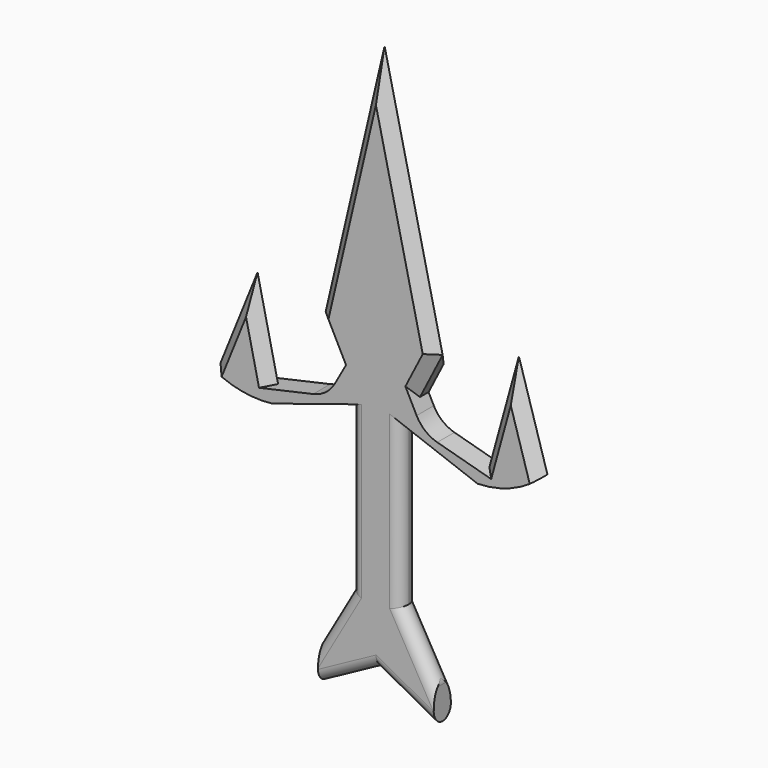
from build123d import *

# Parameters (mm, degrees)
F1_DEPTH      = 3.302
F2_SIZE       = 1.65099
F3_R          = 5.08
F4_T1_DEPTH   = 5.391144251
F4_T6_DEPTH   = 33.5393354473
F4_T12_DEPTH  = 33.5393354473
F4_T18_DEPTH  = 33.5393354473
F4_T24_DEPTH  = 33.5393354473
F4_T30_DEPTH  = 18.415
F4_T35_DEPTH  = 18.415
F4_T40_DEPTH  = 18.415
F4_T45_DEPTH  = 18.415
F4_T50_DEPTH  = 18.415
F4_T55_DEPTH  = 18.415
F4_T60_DEPTH  = 18.415
F4_T65_DEPTH  = 18.415
F4_T71_DEPTH  = 18.415
F4_T75_DEPTH  = 33.5393354473
F4_T82_DEPTH  = 33.5393354473
F4_T86_DEPTH  = 18.415
F4_T93_DEPTH  = 18.415
F4_T97_DEPTH  = 33.5393354473
F4_T104_DEPTH = 33.5393354473
F4_T108_DEPTH = 18.415
F4_T115_DEPTH = 18.415
F4_T119_DEPTH = 18.415
F4_T126_DEPTH = 18.415
F4_T130_DEPTH = 18.415


# Not quite as in the source:
# - a fillet or chamfer that OpenCascade refuses, or shapes differently, is made with other operations: its cross-section is extruded or revolved along the edge and cut away or added
# - a fillet or chamfer is up to 0.001 mm smaller than in the source, because OpenCascade refuses the exact size


with BuildPart() as f1:
    # F0 (on Front) → F1 (new body)
    with BuildSketch(Plane.XZ):
        Polygon((-8.9293484636, -27.2495914251), (-8.9293484636, -32.5835914251), (0, -27.7367021117), (8.9302421297, -32.5819446757), (8.7977098301, -27.2495914251), (3.7441806833, -18.4355433674), (-3.8758193167, -18.4355433674), align=None)
        Polygon((-3.8758193167, 6.8487920798), (-3.8758193167, -18.4355433674), (3.7441806833, -18.4355433674), (3.7441806833, 6.8487920798), (5.4475756045, 10.1900669473), (8.9355429432, 17.0318494737), (0, 55.9675879776), (-9.0671815766, 17.0318494737), (-5.5792142379, 10.1900669473), align=None)
        Polygon((-15.9811842538, 3.0082010134), (-3.8758193167, 6.8487920798), (-5.5792142379, 10.1900669473), (-7.4475542642, 6.8487920798), (-16.3927144946, 4.8489290213), align=None)
        Polygon((5.4475756045, 10.1900669473), (3.7441806833, 6.8487920798), (15.648767343, 2.4249005283), (16.1309282999, 4.1770842273), (7.269941736, 6.61542546), align=None)
        with BuildLine():
            ThreePointArc((-25.2471491773, 4.8381724725), (-20.7595085955, 3.1872557237), (-15.9811842538, 3.0082010134))
            Line((-15.9811842538, 3.0082010134), (-16.3927144946, 4.8489290213))
            Line((-16.3927144946, 4.8489290213), (-19.5505233946, 18.973449431))
            Line((-19.5505233946, 18.973449431), (-25.2471491773, 4.8381724725))
        make_face()
        with BuildLine():
            Line((16.1309282999, 4.1770842273), (15.648767343, 2.4249005283))
            ThreePointArc((15.648767343, 2.4249005283), (20.6670070739, 3.4448326602), (25.0641160129, 6.0694134893))
            Line((25.0641160129, 6.0694134893), (20.6670070739, 20.6612959236))
            Line((20.6670070739, 20.6612959236), (16.1309282999, 4.1770842273))
        make_face()
    extrude(amount=F1_DEPTH)

    # F2 (size 1.651 in the source; OpenCascade refuses exactly that, so slightly less here)
    f2_edges = [f1.edges().sort_by_distance(p)[0] for p in [
        (4.467771, -3.302, 36.499719),
        (-4.533591, -3.302, 36.499719),
        (18.398968, -3.302, 12.41919),
        (22.865562, -3.302, 13.365355),
        (-22.398836, -3.302, 11.905811),
        (-17.971619, -3.302, 11.911189),
        (18.398968, 0, 12.41919),
        (22.865562, 0, 13.365355),
        (-22.398836, 0, 11.905811),
        (-17.971619, 0, 11.911189),
        (7.191559, -3.302, 13.610958),
        (-7.323198, -3.302, 13.610958),
        (4.467771, 0, 36.499719),
        (-4.533591, 0, 36.499719),
    ]]
    chamfer(f2_edges, length=F2_SIZE)

    # F3
    f3_edges = [f1.edges().sort_by_distance(p)[0] for p in [
        (-7.447554, -1.651, 6.848792),
        (7.269942, -1.651, 6.615425),
    ]]
    fillet(f3_edges, radius=F3_R)

    # F4: fillet of radius 1.651 on 13 edges, made by hand

    # F4_s2 → F4_t1 (cut)
    with BuildSketch(Plane.XZ.offset(-1.0445721255)):
        with BuildLine():
            ThreePointArc((8.5898840158, -26.8871146962), (8.7475827705, -27.2636114555), (8.8080914983, -27.6672912803))
            Line((8.8080914983, -27.6672912803), (8.7977098301, -27.2495914251))
            Line((8.7977098301, -27.2495914251), (8.5898840158, -26.8871146962))
        make_face()
    extrude(amount=F4_T1_DEPTH, mode=Mode.SUBTRACT)


with BuildPart() as f4_tool4:
    # F4_s5 → F4_t6 (new body)
    with BuildSketch(Plane.XY.offset(10.9762920798)):
        with BuildLine():
            ThreePointArc((-3.8758193167, -1.651), (-3.3922526125, -2.8184332957), (-2.2248193167, -3.302))
            Line((-2.2248193167, -3.302), (-3.8758193167, -3.302))
            Line((-3.8758193167, -3.302), (-3.8758193167, -1.651))
        make_face()
    extrude(amount=-F4_T6_DEPTH)

    split(bisect_by=Plane(origin=(5.03803687, 0, -2.888555406), x_dir=(0, 1, 0), z_dir=(-0.8675244151, 0, 0.4973946011)), keep=Keep.TOP)

    split(bisect_by=Plane(origin=(-2.3286084058, 0, 7.3396657076), x_dir=(0, 1, 0), z_dir=(0.3024087454, 0, -0.9531783415)), keep=Keep.TOP)


with BuildPart() as f1_1:
    add(f1.part)

    # F4_t3: cut F4_tool4
    add(f4_tool4.part, mode=Mode.SUBTRACT)


with BuildPart() as f4_tool10:
    # F4_s11 → F4_t12 (new body)
    with BuildSketch(Plane.XY.offset(-22.5630433674)):
        with BuildLine():
            ThreePointArc((3.7441806833, -1.651), (3.260613979, -2.8184332957), (2.0931806833, -3.302))
            Line((2.0931806833, -3.302), (3.7441806833, -3.302))
            Line((3.7441806833, -3.302), (3.7441806833, -1.651))
        make_face()
    extrude(amount=F4_T12_DEPTH)

    split(bisect_by=Plane(origin=(2.6905919195, 0, 7.2403186875), x_dir=(0, 1, 0), z_dir=(-0.3483379174, 0, -0.9373690283)), keep=Keep.TOP)

    split(bisect_by=Plane(origin=(-5.1371079227, 0, -2.9453577344), x_dir=(0, 1, 0), z_dir=(0.8675244151, 0, 0.4973946011)), keep=Keep.TOP)


with BuildPart() as f1_2:
    add(f1_1.part)

    # F4_t9: cut F4_tool10
    add(f4_tool10.part, mode=Mode.SUBTRACT)


with BuildPart() as f4_tool16:
    # F4_s17 → F4_t18 (new body)
    with BuildSketch(Plane.XY.offset(10.9762920798)):
        with BuildLine():
            ThreePointArc((-2.2248193167, 0), (-3.3922526125, -0.4835667043), (-3.8758193167, -1.651))
            Line((-3.8758193167, -1.651), (-3.8758193167, 0))
            Line((-3.8758193167, 0), (-2.2248193167, 0))
        make_face()
    extrude(amount=-F4_T18_DEPTH)

    split(bisect_by=Plane(origin=(5.03803687, 0, -2.888555406), x_dir=(0, 1, 0), z_dir=(-0.8675244151, 0, 0.4973946011)), keep=Keep.TOP)

    split(bisect_by=Plane(origin=(-2.3286084058, 0, 7.3396657076), x_dir=(0, 1, 0), z_dir=(0.3024087454, 0, -0.9531783415)), keep=Keep.TOP)


with BuildPart() as f1_3:
    add(f1_2.part)

    # F4_t15: cut F4_tool16
    add(f4_tool16.part, mode=Mode.SUBTRACT)


with BuildPart() as f4_tool22:
    # F4_s23 → F4_t24 (new body)
    with BuildSketch(Plane.XY.offset(-22.5630433674)):
        with BuildLine():
            ThreePointArc((2.0931806833, 0), (3.260613979, -0.4835667043), (3.7441806833, -1.651))
            Line((3.7441806833, -1.651), (3.7441806833, 0))
            Line((3.7441806833, 0), (2.0931806833, 0))
        make_face()
    extrude(amount=F4_T24_DEPTH)

    split(bisect_by=Plane(origin=(2.6905919195, 0, 7.2403186875), x_dir=(0, 1, 0), z_dir=(-0.3483379174, 0, -0.9373690283)), keep=Keep.TOP)

    split(bisect_by=Plane(origin=(-5.1371079227, 0, -2.9453577344), x_dir=(0, 1, 0), z_dir=(0.8675244151, 0, 0.4973946011)), keep=Keep.TOP)


with BuildPart() as f1_4:
    add(f1_3.part)

    # F4_t21: cut F4_tool22
    add(f4_tool22.part, mode=Mode.SUBTRACT)


with BuildPart() as f4_tool28:
    # F4_s29 → F4_t30 (new body)
    with BuildSketch(Plane(origin=(-6.8608599708, 0, -11.966280938), x_dir=(0, 1, 0), z_dir=(-0.4973946011, 0, -0.8675244151))):
        with BuildLine():
            ThreePointArc((0, 7.4583718528), (-0.4835667043, 6.2909385571), (-1.651, 5.8073718528))
            Line((-1.651, 5.8073718528), (0, 5.8073718528))
            Line((0, 5.8073718528), (0, 7.4583718528))
        make_face()
    extrude(amount=F4_T30_DEPTH)

    split(bisect_by=Plane.YZ.offset(-3.8758193167), keep=Keep.BOTTOM)


with BuildPart() as f1_5:
    add(f1_4.part)

    # F4_t27: cut F4_tool28
    add(f4_tool28.part, mode=Mode.SUBTRACT)


with BuildPart() as f4_tool33:
    # F4_s34 → F4_t35 (new body)
    with BuildSketch(Plane(origin=(-6.8608599708, 0, -11.966280938), x_dir=(0, 1, 0), z_dir=(-0.4973946011, 0, -0.8675244151))):
        with BuildLine():
            ThreePointArc((-1.651, 5.8073718528), (-2.8184332957, 6.2909385571), (-3.302, 7.4583718528))
            Line((-3.302, 7.4583718528), (-3.302, 5.8073718528))
            Line((-3.302, 5.8073718528), (-1.651, 5.8073718528))
        make_face()
    extrude(amount=F4_T35_DEPTH)

    split(bisect_by=Plane.YZ.offset(-3.8758193167), keep=Keep.BOTTOM)


with BuildPart() as f1_6:
    add(f1_5.part)

    # F4_t32: cut F4_tool33
    add(f4_tool33.part, mode=Mode.SUBTRACT)


with BuildPart() as f4_tool38:
    # F4_s39 → F4_t40 (new body)
    with BuildSketch(Plane(origin=(-24.1861080645, 0, -13.1283250048), x_dir=(0, 1, 0), z_dir=(0.8788728803, 0, 0.4770560348))):
        with BuildLine():
            ThreePointArc((0, -22.7260352741), (-0.4835667043, -23.8934685698), (-1.651, -24.3770352741))
            Line((-1.651, -24.3770352741), (0, -24.3770352741))
            Line((0, -24.3770352741), (0, -22.7260352741))
        make_face()
    extrude(amount=F4_T40_DEPTH)

    split(bisect_by=Plane(origin=(-11.6264241962, 0, -21.4286037908), x_dir=(0, 1, 0), z_dir=(-0.4768939532, 0, -0.8789608395)), keep=Keep.TOP)


with BuildPart() as f1_7:
    add(f1_6.part)

    # F4_t37: cut F4_tool38
    add(f4_tool38.part, mode=Mode.SUBTRACT)


with BuildPart() as f4_tool43:
    # F4_s44 → F4_t45 (new body)
    with BuildSketch(Plane(origin=(-24.1861080645, 0, -13.1283250048), x_dir=(0, 1, 0), z_dir=(0.8788728803, 0, 0.4770560348))):
        with BuildLine():
            ThreePointArc((-1.651, -24.3770352741), (-2.8184332957, -23.8934685698), (-3.302, -22.7260352741))
            Line((-3.302, -22.7260352741), (-3.302, -24.3770352741))
            Line((-3.302, -24.3770352741), (-1.651, -24.3770352741))
        make_face()
    extrude(amount=F4_T45_DEPTH)

    split(bisect_by=Plane(origin=(-11.6264241962, 0, -21.4286037908), x_dir=(0, 1, 0), z_dir=(-0.4768939532, 0, -0.8789608395)), keep=Keep.TOP)


with BuildPart() as f1_8:
    add(f1_7.part)

    # F4_t42: cut F4_tool43
    add(f4_tool43.part, mode=Mode.SUBTRACT)


with BuildPart() as f4_tool48:
    # F4_s49 → F4_t50 (new body)
    with BuildSketch(Plane(origin=(15.9878139687, 0, -27.8849407141), x_dir=(0, 1, 0), z_dir=(-0.4973946011, 0, 0.8675244151))):
        with BuildLine():
            ThreePointArc((-1.651, 5.9215715813), (-2.8184332957, 6.4051382856), (-3.302, 7.5725715813))
            Line((-3.302, 7.5725715813), (-3.302, 5.9215715813))
            Line((-3.302, 5.9215715813), (-1.651, 5.9215715813))
        make_face()
    extrude(amount=F4_T50_DEPTH)

    split(bisect_by=Plane.YZ.offset(3.7441806833), keep=Keep.TOP)


with BuildPart() as f1_9:
    add(f1_8.part)

    # F4_t47: cut F4_tool48
    add(f4_tool48.part, mode=Mode.SUBTRACT)


with BuildPart() as f4_tool53:
    # F4_s54 → F4_t55 (new body)
    with BuildSketch(Plane(origin=(15.9878139687, 0, -27.8849407141), x_dir=(0, 1, 0), z_dir=(-0.4973946011, 0, 0.8675244151))):
        with BuildLine():
            ThreePointArc((0, 7.5725715813), (-0.4835667043, 6.4051382856), (-1.651, 5.9215715813))
            Line((-1.651, 5.9215715813), (0, 5.9215715813))
            Line((0, 5.9215715813), (0, 7.5725715813))
        make_face()
    extrude(amount=F4_T55_DEPTH)

    split(bisect_by=Plane.YZ.offset(3.7441806833), keep=Keep.TOP)


with BuildPart() as f1_10:
    add(f1_9.part)

    # F4_t52: cut F4_tool53
    add(f4_tool53.part, mode=Mode.SUBTRACT)


with BuildPart() as f4_tool58:
    # F4_s59 → F4_t60 (new body)
    with BuildSketch(Plane(origin=(7.998513331, 0, -4.3397185292), x_dir=(0, 1, 0), z_dir=(0.8789608395, 0, -0.4768939532))):
        with BuildLine():
            ThreePointArc((0, -22.7284749742), (-0.4835667043, -23.8959082699), (-1.651, -24.3794749742))
            Line((-1.651, -24.3794749742), (0, -24.3794749742))
            Line((0, -24.3794749742), (0, -22.7284749742))
        make_face()
    extrude(amount=F4_T60_DEPTH)

    split(bisect_by=Plane(origin=(11.6292117876, 0, -21.4243152038), x_dir=(0, 1, 0), z_dir=(0.4770560348, 0, -0.8788728803)), keep=Keep.TOP)


with BuildPart() as f1_11:
    add(f1_10.part)

    # F4_t57: cut F4_tool58
    add(f4_tool58.part, mode=Mode.SUBTRACT)


with BuildPart() as f4_tool63:
    # F4_s64 → F4_t65 (new body)
    with BuildSketch(Plane(origin=(7.998513331, 0, -4.3397185292), x_dir=(0, 1, 0), z_dir=(0.8789608395, 0, -0.4768939532))):
        with BuildLine():
            ThreePointArc((-1.651, -24.3794749742), (-2.8184332957, -23.8959082699), (-3.302, -22.7284749742))
            Line((-3.302, -22.7284749742), (-3.302, -24.3794749742))
            Line((-3.302, -24.3794749742), (-1.651, -24.3794749742))
        make_face()
    extrude(amount=F4_T65_DEPTH)

    split(bisect_by=Plane(origin=(11.6292117876, 0, -21.4243152038), x_dir=(0, 1, 0), z_dir=(0.4770560348, 0, -0.8788728803)), keep=Keep.TOP)


with BuildPart() as f1_12:
    add(f1_11.part)

    # F4_t62: cut F4_tool63
    add(f4_tool63.part, mode=Mode.SUBTRACT)


with BuildPart() as f4_tool69:
    # F4_s70 → F4_t71 (new body)
    with BuildSketch(Plane(origin=(-6.8608599708, 0, -11.966280938), x_dir=(0, 1, 0), z_dir=(-0.4973946011, 0, -0.8675244151))):
        with BuildLine():
            ThreePointArc((-1.651, 5.8073718528), (-2.8184332957, 6.2909385571), (-3.302, 7.4583718528))
            Line((-3.302, 7.4583718528), (-3.302, 5.8073718528))
            Line((-3.302, 5.8073718528), (-1.651, 5.8073718528))
        make_face()
    extrude(amount=F4_T71_DEPTH)

    split(bisect_by=Plane.YZ.offset(-3.8758193167), keep=Keep.TOP)


with BuildPart() as f4_tool73:
    # F4_s74 → F4_t75 (new body)
    with BuildSketch(Plane.XY.offset(10.9762920798)):
        with BuildLine():
            ThreePointArc((-3.8758193167, -1.651), (-3.3922526125, -2.8184332957), (-2.2248193167, -3.302))
            Line((-2.2248193167, -3.302), (-3.8758193167, -3.302))
            Line((-3.8758193167, -3.302), (-3.8758193167, -1.651))
        make_face()
    extrude(amount=-F4_T75_DEPTH)

    split(bisect_by=Plane(origin=(5.03803687, 0, -2.888555406), x_dir=(0, 1, 0), z_dir=(0.8675244151, 0, -0.4973946011)), keep=Keep.TOP)


with BuildPart() as f4_tool69_1:
    add(f4_tool69.part)

    # F4_t77: intersect F4_tool73
    add(f4_tool73.part, mode=Mode.INTERSECT)


with BuildPart() as f1_13:
    add(f1_12.part)

    # F4_t67: cut F4_tool69
    add(f4_tool69_1.part, mode=Mode.SUBTRACT)


with BuildPart() as f4_tool80:
    # F4_s81 → F4_t82 (new body)
    with BuildSketch(Plane.XY.offset(-22.5630433674)):
        with BuildLine():
            ThreePointArc((3.7441806833, -1.651), (3.260613979, -2.8184332957), (2.0931806833, -3.302))
            Line((2.0931806833, -3.302), (3.7441806833, -3.302))
            Line((3.7441806833, -3.302), (3.7441806833, -1.651))
        make_face()
    extrude(amount=F4_T82_DEPTH)

    split(bisect_by=Plane(origin=(-5.1371079227, 0, -2.9453577344), x_dir=(0, 1, 0), z_dir=(-0.8675244151, 0, -0.4973946011)), keep=Keep.TOP)


with BuildPart() as f4_tool84:
    # F4_s85 → F4_t86 (new body)
    with BuildSketch(Plane(origin=(15.9878139687, 0, -27.8849407141), x_dir=(0, 1, 0), z_dir=(-0.4973946011, 0, 0.8675244151))):
        with BuildLine():
            ThreePointArc((-1.651, 5.9215715813), (-2.8184332957, 6.4051382856), (-3.302, 7.5725715813))
            Line((-3.302, 7.5725715813), (-3.302, 5.9215715813))
            Line((-3.302, 5.9215715813), (-1.651, 5.9215715813))
        make_face()
    extrude(amount=F4_T86_DEPTH)

    split(bisect_by=Plane.YZ.offset(3.7441806833), keep=Keep.BOTTOM)


with BuildPart() as f4_tool80_1:
    add(f4_tool80.part)

    # F4_t88: intersect F4_tool84
    add(f4_tool84.part, mode=Mode.INTERSECT)


with BuildPart() as f1_14:
    add(f1_13.part)

    # F4_t78: cut F4_tool80
    add(f4_tool80_1.part, mode=Mode.SUBTRACT)


with BuildPart() as f4_tool91:
    # F4_s92 → F4_t93 (new body)
    with BuildSketch(Plane(origin=(-6.8608599708, 0, -11.966280938), x_dir=(0, 1, 0), z_dir=(-0.4973946011, 0, -0.8675244151))):
        with BuildLine():
            ThreePointArc((0, 7.4583718528), (-0.4835667043, 6.2909385571), (-1.651, 5.8073718528))
            Line((-1.651, 5.8073718528), (0, 5.8073718528))
            Line((0, 5.8073718528), (0, 7.4583718528))
        make_face()
    extrude(amount=F4_T93_DEPTH)

    split(bisect_by=Plane.YZ.offset(-3.8758193167), keep=Keep.TOP)


with BuildPart() as f4_tool95:
    # F4_s96 → F4_t97 (new body)
    with BuildSketch(Plane.XY.offset(10.9762920798)):
        with BuildLine():
            ThreePointArc((-2.2248193167, 0), (-3.3922526125, -0.4835667043), (-3.8758193167, -1.651))
            Line((-3.8758193167, -1.651), (-3.8758193167, 0))
            Line((-3.8758193167, 0), (-2.2248193167, 0))
        make_face()
    extrude(amount=-F4_T97_DEPTH)

    split(bisect_by=Plane(origin=(5.03803687, 0, -2.888555406), x_dir=(0, 1, 0), z_dir=(0.8675244151, 0, -0.4973946011)), keep=Keep.TOP)


with BuildPart() as f4_tool91_1:
    add(f4_tool91.part)

    # F4_t99: intersect F4_tool95
    add(f4_tool95.part, mode=Mode.INTERSECT)


with BuildPart() as f1_15:
    add(f1_14.part)

    # F4_t89: cut F4_tool91
    add(f4_tool91_1.part, mode=Mode.SUBTRACT)


with BuildPart() as f4_tool102:
    # F4_s103 → F4_t104 (new body)
    with BuildSketch(Plane.XY.offset(-22.5630433674)):
        with BuildLine():
            ThreePointArc((2.0931806833, 0), (3.260613979, -0.4835667043), (3.7441806833, -1.651))
            Line((3.7441806833, -1.651), (3.7441806833, 0))
            Line((3.7441806833, 0), (2.0931806833, 0))
        make_face()
    extrude(amount=F4_T104_DEPTH)

    split(bisect_by=Plane(origin=(-5.1371079227, 0, -2.9453577344), x_dir=(0, 1, 0), z_dir=(-0.8675244151, 0, -0.4973946011)), keep=Keep.TOP)


with BuildPart() as f4_tool106:
    # F4_s107 → F4_t108 (new body)
    with BuildSketch(Plane(origin=(15.9878139687, 0, -27.8849407141), x_dir=(0, 1, 0), z_dir=(-0.4973946011, 0, 0.8675244151))):
        with BuildLine():
            ThreePointArc((0, 7.5725715813), (-0.4835667043, 6.4051382856), (-1.651, 5.9215715813))
            Line((-1.651, 5.9215715813), (0, 5.9215715813))
            Line((0, 5.9215715813), (0, 7.5725715813))
        make_face()
    extrude(amount=F4_T108_DEPTH)

    split(bisect_by=Plane.YZ.offset(3.7441806833), keep=Keep.BOTTOM)


with BuildPart() as f4_tool102_1:
    add(f4_tool102.part)

    # F4_t110: intersect F4_tool106
    add(f4_tool106.part, mode=Mode.INTERSECT)


with BuildPart() as f1_16:
    add(f1_15.part)

    # F4_t100: cut F4_tool102
    add(f4_tool102_1.part, mode=Mode.SUBTRACT)


with BuildPart() as f4_tool113:
    # F4_s114 → F4_t115 (new body)
    with BuildSketch(Plane(origin=(7.998513331, 0, -4.3397185292), x_dir=(0, 1, 0), z_dir=(0.8789608395, 0, -0.4768939532))):
        with BuildLine():
            ThreePointArc((0, -22.7284749742), (-0.4835667043, -23.8959082699), (-1.651, -24.3794749742))
            Line((-1.651, -24.3794749742), (0, -24.3794749742))
            Line((0, -24.3794749742), (0, -22.7284749742))
        make_face()
    extrude(amount=F4_T115_DEPTH)

    split(bisect_by=Plane(origin=(11.6292117876, 0, -21.4243152038), x_dir=(0, 1, 0), z_dir=(-0.4770560348, 0, 0.8788728803)), keep=Keep.TOP)


with BuildPart() as f4_tool117:
    # F4_s118 → F4_t119 (new body)
    with BuildSketch(Plane(origin=(-24.1861080645, 0, -13.1283250048), x_dir=(0, 1, 0), z_dir=(0.8788728803, 0, 0.4770560348))):
        with BuildLine():
            ThreePointArc((0, -22.7260352741), (-0.4835667043, -23.8934685698), (-1.651, -24.3770352741))
            Line((-1.651, -24.3770352741), (0, -24.3770352741))
            Line((0, -24.3770352741), (0, -22.7260352741))
        make_face()
    extrude(amount=F4_T119_DEPTH)

    split(bisect_by=Plane(origin=(-11.6264241962, 0, -21.4286037908), x_dir=(0, 1, 0), z_dir=(0.4768939532, 0, 0.8789608395)), keep=Keep.TOP)


with BuildPart() as f4_tool113_1:
    add(f4_tool113.part)

    # F4_t121: intersect F4_tool117
    add(f4_tool117.part, mode=Mode.INTERSECT)


with BuildPart() as f1_17:
    add(f1_16.part)

    # F4_t111: cut F4_tool113
    add(f4_tool113_1.part, mode=Mode.SUBTRACT)


with BuildPart() as f4_tool124:
    # F4_s125 → F4_t126 (new body)
    with BuildSketch(Plane(origin=(7.998513331, 0, -4.3397185292), x_dir=(0, 1, 0), z_dir=(0.8789608395, 0, -0.4768939532))):
        with BuildLine():
            ThreePointArc((-1.651, -24.3794749742), (-2.8184332957, -23.8959082699), (-3.302, -22.7284749742))
            Line((-3.302, -22.7284749742), (-3.302, -24.3794749742))
            Line((-3.302, -24.3794749742), (-1.651, -24.3794749742))
        make_face()
    extrude(amount=F4_T126_DEPTH)

    split(bisect_by=Plane(origin=(11.6292117876, 0, -21.4243152038), x_dir=(0, 1, 0), z_dir=(-0.4770560348, 0, 0.8788728803)), keep=Keep.TOP)


with BuildPart() as f4_tool128:
    # F4_s129 → F4_t130 (new body)
    with BuildSketch(Plane(origin=(-24.1861080645, 0, -13.1283250048), x_dir=(0, 1, 0), z_dir=(0.8788728803, 0, 0.4770560348))):
        with BuildLine():
            ThreePointArc((-1.651, -24.3770352741), (-2.8184332957, -23.8934685698), (-3.302, -22.7260352741))
            Line((-3.302, -22.7260352741), (-3.302, -24.3770352741))
            Line((-3.302, -24.3770352741), (-1.651, -24.3770352741))
        make_face()
    extrude(amount=F4_T130_DEPTH)

    split(bisect_by=Plane(origin=(-11.6264241962, 0, -21.4286037908), x_dir=(0, 1, 0), z_dir=(0.4768939532, 0, 0.8789608395)), keep=Keep.TOP)


with BuildPart() as f4_tool124_1:
    add(f4_tool124.part)

    # F4_t132: intersect F4_tool128
    add(f4_tool128.part, mode=Mode.INTERSECT)


with BuildPart() as f1_18:
    add(f1_17.part)

    # F4_t122: cut F4_tool124
    add(f4_tool124_1.part, mode=Mode.SUBTRACT)


solid = f1_18.part
